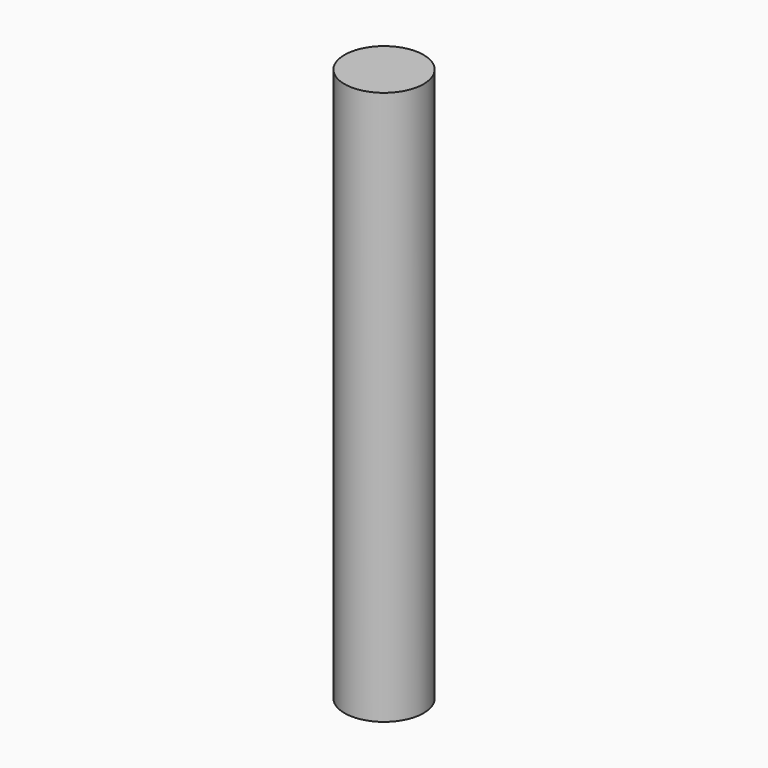
from build123d import *

# Parameters (mm, degrees)
F1_R     = 6.35
F2_DEPTH = 88.9


# Not quite as in the source:
# - a variable given as a bare number and used for a length is read in inches; the dataset says mm whatever the document's units were


with BuildPart() as f2:
    # F1 (on Top) → F2 (new body)
    with BuildSketch(Plane.XY):
        Circle(F1_R)
    extrude(amount=F2_DEPTH)


solid = f2.part
